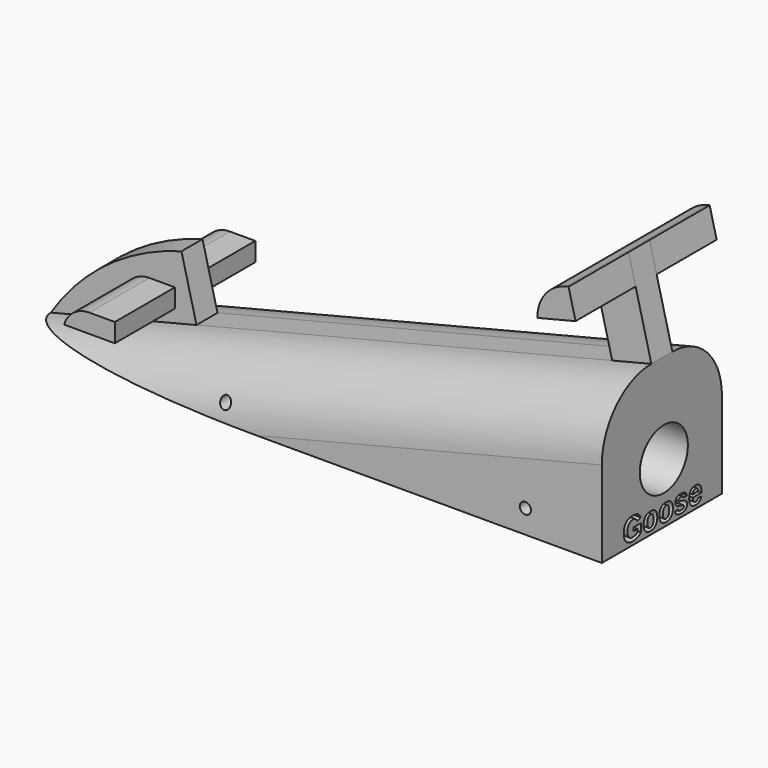
from build123d import *

# Parameters (mm, degrees)
F1_DEPTH      = 50.8
F2_R          = 10.16
F3_DEPTH      = 52.07
F4_R          = 20.955
F5_W          = 50.8
F5_H          = 8.89
F6_DEPTH      = 20.955
F7_T1_DEPTH   = 271.3033178309
F8_W          = 17.145
F8_H          = 6.35
F9_DEPTH      = 25.4
F9_DEPTH_BACK = 34.036
F10_T1_DEPTH  = 46.6985474857
F10_T3_DEPTH  = 46.4445474857
F10_T8_DEPTH  = 67.9970949714
F10_T13_DEPTH = 67.7430949714
F12_D         = 3.81
F13_TEXT_SIZE = 10.8414646497
F14_DEPTH     = 12.7
F15_W         = 13.6662203978
F15_H         = 8.89
F16_DEPTH     = 31.75
F18_DEPTH     = 25.4
F20_DEPTH     = 25.4
F21_T1_DEPTH  = 123.19


# Not quite as in the source:
# - a fillet or chamfer that OpenCascade refuses, or shapes differently, is made with other operations: its cross-section is extruded or revolved along the edge and cut away or added
# - Text() gives the source's letters only with a copy of the font that has no kerning and outlines rounded to 1/6400 em; it was checked with that copy


with BuildPart() as f1:
    # F0 (on Front) → F1 (new body)
    with BuildSketch(Plane.XZ):
        Polygon((101.9375402447, 50.8), (-101.2624597553, 0), (101.9375402447, 0), align=None)
    extrude(amount=F1_DEPTH)

    # F2 (on face) → F3 (cut)
    with BuildSketch(Plane.YZ.offset(101.9375402447)):
        with Locations((-24.5673861355, 20.32)):
            Circle(F2_R)
    extrude(amount=-F3_DEPTH, mode=Mode.SUBTRACT)

    # F4
    f4_edges = [f1.edges().sort_by_distance(p)[0] for p in [
        (0.33754, -50.8, 25.4),
        (0.33754, 0, 25.4),
    ]]
    fillet(f4_edges, radius=F4_R)

    # F5 (on face) → F6 (join)
    with BuildSketch(Plane(origin=(-5.9566152797, 0, 23.8264611189), x_dir=(0.9701425001, 0, 0.242535625), z_dir=(-0.242535625, 0, 0.9701425001))):
        with Locations((-72.8390158778, -25.4)):
            Rectangle(F5_W, F5_H)
    extrude(amount=F6_DEPTH)

    # F7: fillet of radius 76.2 on 1 edges, made by hand

    # F7_s2 → F7_t1 (cut)
    with BuildSketch(Plane.XZ.offset(-110.2516589154)):
        with BuildLine():
            ThreePointArc((-55.4291313315, 33.0582517021), (-81.5236542055, 20.9350406301), (-101.2624597553, 0))
            Line((-101.2624597553, 0), (-106.3447937779, 20.3293360905))
            Line((-106.3447937779, 20.3293360905), (-55.4291313315, 33.0582517021))
        make_face()
    extrude(amount=F7_T1_DEPTH, mode=Mode.SUBTRACT)

    # F8 (on face) → F9 (join, two sides)
    with BuildSketch(Plane.XZ.offset(29.845)) as f9_sk:
        with Locations((-67.8719580173, 17.9937942865)):
            Rectangle(F8_W, F8_H)
    extrude(amount=F9_DEPTH)
    extrude(f9_sk.sketch, amount=-F9_DEPTH_BACK)

    # F10: fillet of radius 8.89 on 2 edges, made by hand

    # F10_s2 → F10_t1 (cut)
    with BuildSketch(Plane.XZ.offset(29.845)):
        with BuildLine():
            ThreePointArc((-76.4444580173, 14.8187942865), (-73.2378301916, 19.4066516083), (-67.9250390231, 21.1687942865))
            Line((-67.9250390231, 21.1687942865), (-76.4444580173, 21.1687942865))
            Line((-76.4444580173, 21.1687942865), (-76.4444580173, 14.8187942865))
        make_face()
    extrude(amount=F10_T1_DEPTH, mode=Mode.SUBTRACT)

    # F10_s4 → F10_t3 (cut)
    with BuildSketch(Plane.XZ.offset(-25.4895474857)):
        with BuildLine():
            ThreePointArc((-76.4444580173, 14.8187942865), (-73.2378301916, 19.4066516083), (-67.9250390231, 21.1687942865))
            Line((-67.9250390231, 21.1687942865), (-76.4444580173, 21.1687942865))
            Line((-76.4444580173, 21.1687942865), (-76.4444580173, 14.8187942865))
        make_face()
    extrude(amount=F10_T3_DEPTH, mode=Mode.SUBTRACT)


with BuildPart() as f10_tool6:
    # F10_s7 → F10_t8 (new body)
    with BuildSketch(Plane.XZ.offset(8.5464525143)):
        with BuildLine():
            ThreePointArc((-76.4444580173, 14.8187942865), (-73.2378301916, 19.4066516083), (-67.9250390231, 21.1687942865))
            Line((-67.9250390231, 21.1687942865), (-76.4444580173, 21.1687942865))
            Line((-76.4444580173, 21.1687942865), (-76.4444580173, 14.8187942865))
        make_face()
    extrude(amount=F10_T8_DEPTH)

    split(bisect_by=Plane.XZ.offset(20.955), keep=Keep.BOTTOM)


with BuildPart() as f1_1:
    add(f1.part)

    # F10_t5: cut F10_tool6
    add(f10_tool6.part, mode=Mode.SUBTRACT)


with BuildPart() as f10_tool11:
    # F10_s12 → F10_t13 (new body)
    with BuildSketch(Plane.XZ.offset(-25.4895474857)):
        with BuildLine():
            ThreePointArc((-76.4444580173, 14.8187942865), (-73.2378301916, 19.4066516083), (-67.9250390231, 21.1687942865))
            Line((-67.9250390231, 21.1687942865), (-76.4444580173, 21.1687942865))
            Line((-76.4444580173, 21.1687942865), (-76.4444580173, 14.8187942865))
        make_face()
    extrude(amount=F10_T13_DEPTH)

    split(bisect_by=Plane.XZ.offset(29.845), keep=Keep.TOP)


with BuildPart() as f1_2:
    add(f1_1.part)

    # F10_t10: cut F10_tool11
    add(f10_tool11.part, mode=Mode.SUBTRACT)

    # F12 (through all)
    with Locations(Plane.XZ.offset(50.8)):
        with Locations((-26.6350358725, 5.3167096339), (76.0682374239, 7.910227403)):
            Hole(F12_D / 2)

    # F13 (on face) → F14 (cut)
    with BuildSketch(Plane.YZ.offset(101.9375402447)):
        with Locations((-41.9742926024, 1.2497087009)):
            Text('Goose', F13_TEXT_SIZE, font='Arimo', font_style=FontStyle.BOLD, text_align=(TextAlign.LEFT, TextAlign.BOTTOM))
    extrude(amount=-F14_DEPTH, mode=Mode.SUBTRACT)

    # F15 (on face) → F16 (join)
    with BuildSketch(Plane(origin=(-5.9566152797, 0, 23.8264611189), x_dir=(0.9701425001, 0, 0.242535625), z_dir=(-0.242535625, 0, 0.9701425001))):
        with Locations((104.3816397046, -25.4)):
            Rectangle(F15_W, F15_H)
    extrude(amount=F16_DEPTH)

    # F17 (on face) → F18 (join)
    with BuildSketch(Plane(origin=(0, -20.955, 0), x_dir=(-1, 0, 0), z_dir=(0, 1, 0))):
        Polygon((-80.9788529256, 78.2874790735), (-94.2370341498, 81.6020243796), (-96.6087900271, 72.1150008707), (-83.3506088028, 68.8004555646), align=None)
    extrude(amount=F18_DEPTH)

    # F19 (on face) → F20 (join)
    with BuildSketch(Plane.XZ.offset(29.845)):
        Polygon((94.2370341498, 81.6020243796), (80.9788529256, 78.2874790735), (83.3506088028, 68.8004555646), (96.6087900271, 72.1150008707), align=None)
    extrude(amount=F20_DEPTH)

    # F21: fillet of radius 12.7 on 1 edges, made by hand

    # F21_s2 → F21_t1 (cut)
    with BuildSketch(Plane.XZ.offset(-36.195)):
        with BuildLine():
            ThreePointArc((84.0590553635, 65.9666693217), (85.4897049588, 75.5809678536), (93.2996626774, 81.3676815115))
            Line((93.2996626774, 81.3676815115), (80.9788529256, 78.2874790735))
            Line((80.9788529256, 78.2874790735), (84.0590553635, 65.9666693217))
        make_face()
    extrude(amount=F21_T1_DEPTH, mode=Mode.SUBTRACT)


solid = f1_2.part
